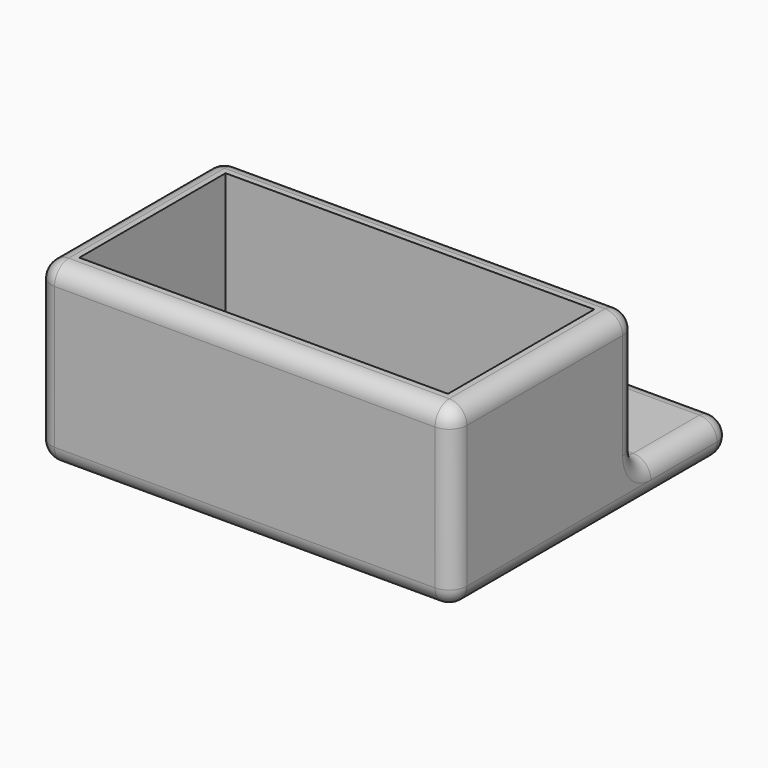
from build123d import *

# Parameters (mm, degrees)
F0_W     = 35.25
F0_H     = 19.5
F0_W_2   = 31.25
F0_H_2   = 15.5
F1_DEPTH = 15
F0_H_3   = 10
F0_R     = 2
F2_DEPTH = 3
F3_R     = 1.49999


# Not quite as in the source:
# - a fillet or chamfer is up to 0.001 mm smaller than in the source, because OpenCascade refuses the exact size


with BuildPart() as f1:
    # F0 (on Top) → F1 (new body)
    with BuildSketch(Plane.XY):
        Rectangle(F0_W, F0_H)
        Rectangle(F0_W_2, F0_H_2, mode=Mode.SUBTRACT)
    extrude(amount=F1_DEPTH)

    # F0 (on Top) → F2 (join)
    with BuildSketch(Plane.XY):
        Rectangle(F0_W_2, F0_H_2)
        with Locations((0, 14.75)):
            Rectangle(F0_W, F0_H_3)
        with Locations((-8, 14.75)):
            Circle(F0_R, mode=Mode.SUBTRACT)
        with Locations((8, 14.75)):
            Circle(F0_R, mode=Mode.SUBTRACT)
    extrude(amount=F2_DEPTH)

    # F3 (radius 1.5 in the source; OpenCascade refuses exactly that, so slightly less here)
    f3_edges = [f1.edges().sort_by_distance(p)[0] for p in [
        (-17.625, 14.75, 3),
        (0, 9.75, 3),
        (17.625, 14.75, 3),
        (0, 19.75, 3),
        (-10, 14.75, 3),
        (6, 14.75, 3),
        (0, -9.75, 0),
        (17.625, 5, 0),
        (0, 19.75, 0),
        (-17.625, 5, 0),
        (6, 14.75, 0),
        (-10, 14.75, 0),
        (-17.625, 9.75, 9),
        (-17.625, 0, 15),
        (-17.625, -9.75, 7.5),
        (-17.625, 19.75, 1.5),
        (17.625, -9.75, 7.5),
        (17.625, 0, 15),
        (17.625, 9.75, 9),
        (17.625, 19.75, 1.5),
        (0, -9.75, 15),
        (0, 9.75, 15),
    ]]
    fillet(f3_edges, radius=F3_R)


solid = f1.part
